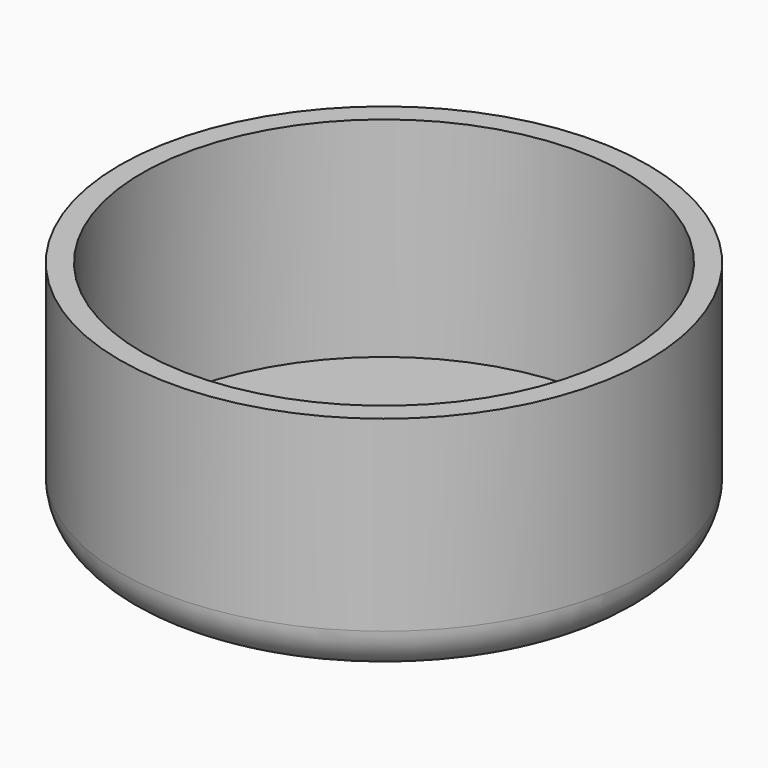
from build123d import *

# Parameters (mm, degrees)
F0_R     = 12
F0_R_2   = 11
F1_DEPTH = 10.5
F2_DEPTH = 1
F3_R     = 6.5
F4_DEPTH = 25


# Not quite as in the source:
# - a fillet or chamfer that OpenCascade refuses, or shapes differently, is made with other operations: its cross-section is extruded or revolved along the edge and cut away or added


with BuildPart() as f1:
    # F0 (on Top) → F1 (new body)
    with BuildSketch(Plane.XY):
        Circle(F0_R)
        Circle(F0_R_2, mode=Mode.SUBTRACT)
    extrude(amount=F1_DEPTH)

    # F0 (on Top) → F2 (join)
    with BuildSketch(Plane.XY):
        Circle(F0_R_2)
    extrude(amount=F2_DEPTH)

    # F3 (on face) → F4 (cut)
    with BuildSketch(Plane.XY):
        Circle(F3_R)
    extrude(amount=F4_DEPTH, mode=Mode.SUBTRACT)

    # F5: fillet of radius 2 on 2 edges, made by hand

    # F5_s1 → F5_t2 (revolve, cut)
    with BuildSketch(Plane.XZ):
        with BuildLine():
            ThreePointArc((12, 2), (11.4142135624, 0.5857864376), (10, 0))
            Line((10, 0), (12, 0))
            Line((12, 0), (12, 2))
        make_face()
    revolve(axis=Axis((0, 0, 0), (0, 0, 1)), mode=Mode.SUBTRACT)

    # F5_s3 → F5_t4 (revolve, cut)
    with BuildSketch(Plane.XZ):
        with BuildLine():
            ThreePointArc((8.2320508076, 0), (7.2320508076, 0.2679491924), (6.5, 1))
            Line((6.5, 1), (6.5, 0))
            Line((6.5, 0), (8.2320508076, 0))
        make_face()
    revolve(axis=Axis((0, 0, 0), (0, 0, 1)), mode=Mode.SUBTRACT)


solid = f1.part
